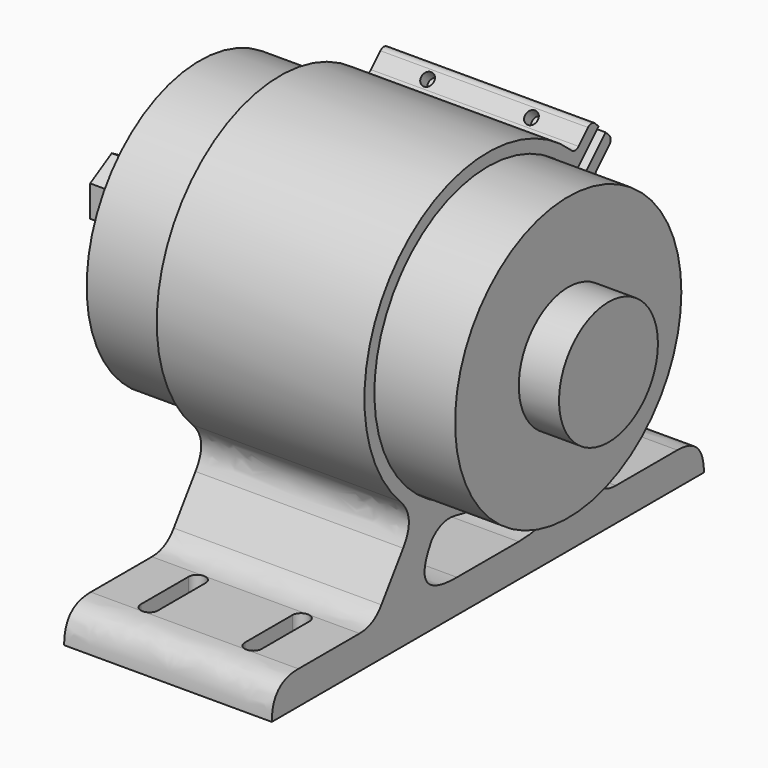
from build123d import *

# Parameters (mm, degrees)
F0_R         = 34.05
F1_DEPTH     = 44.35
F2_R         = 14.875
F3_DEPTH     = 9.7
F4_R         = 6
F5_DEPTH     = 9.55
F6_R         = 12.5
F7_DEPTH     = 2.8
F9_DEPTH     = 8.85
F10_DEPTH    = 25
F11_T1_DEPTH = 50
F11_T3_DEPTH = 90
F13_DEPTH    = 8.0010001
F14_R        = 1.55
F15_DEPTH    = 86.3860158555
F16_R        = 1.5


# Not quite as in the source:
# - a fillet or chamfer that OpenCascade refuses, or shapes differently, is made with other operations: its cross-section is extruded or revolved along the edge and cut away or added


with BuildPart() as f1:
    # F0 (on Right) → F1 (new body, symmetric)
    with BuildSketch(Plane.YZ):
        Circle(F0_R)
    extrude(amount=F1_DEPTH, both=True)

    # F2 (on face) → F3 (join)
    with BuildSketch(Plane.YZ.offset(44.35)):
        Circle(F2_R)
    extrude(amount=F3_DEPTH)

    # F4 (on face) → F5 (join)
    with BuildSketch(Plane(origin=(-44.35, 0, 0), x_dir=(0, -1, 0), z_dir=(-1, 0, 0))):
        Circle(F4_R)
    extrude(amount=F5_DEPTH)


with BuildPart() as f7:
    # F6 (on face) → F7 (new body)
    with BuildSketch(Plane(origin=(-53.9, 0, 0), x_dir=(0, -1, 0), z_dir=(-1, 0, 0))):
        Circle(F6_R)
    extrude(amount=F7_DEPTH)


with BuildPart() as f9:
    # F8 (on face) → F9 (new body)
    with BuildSketch(Plane(origin=(-56.7, 0, 0), x_dir=(0, -1, 0), z_dir=(-1, 0, 0))):
        Polygon((6.5, 3.7527767497), (0, 7.5055534995), (-6.5, 3.7527767497), (-6.5, -3.7527767497), (0, -7.5055534995), (6.5, -3.7527767497), align=None)
    extrude(amount=F9_DEPTH)


with BuildPart() as f10:
    # F0 (on Right) → F10 (new body, symmetric)
    with BuildSketch(Plane.YZ):
        with BuildLine():
            ThreePointArc((28.0146918209, 19.5294531972), (-27.1218147701, -20.7516183363), (26.1756598689, 21.9330191818))
            Line((26.1756598689, 21.9330191818), (33.3400847329, 29.0974440458))
            Line((33.3400847329, 29.0974440458), (31.2187643894, 31.2187643894))
            Line((31.2187643894, 31.2187643894), (26.2690169211, 26.2690169211))
            ThreePointArc((26.2690169211, 26.2690169211), (-28.4585510619, 23.8795596999), (-21.3083646104, -30.4314984453))
            Line((-21.3083646104, -30.4314984453), (-34.415200503, -49.15))
            Line((-34.415200503, -49.15), (-65.0168608087, -49.15))
            Line((-65.0168608087, -49.15), (-65.0168608087, -57.15))
            Line((-65.0168608087, -57.15), (-40.0168608087, -57.15))
            Line((-40.0168608087, -57.15), (40.0168608087, -57.15))
            Line((40.0168608087, -57.15), (65.0168608087, -57.15))
            Line((65.0168608087, -57.15), (65.0168608087, -49.15))
            Line((65.0168608087, -49.15), (34.415200503, -49.15))
            Line((34.415200503, -49.15), (21.3083646104, -30.4314984453))
            ThreePointArc((21.3083646104, -30.4314984453), (36.3368391247, -7.7302407742), (31.8504204749, 19.1225839147))
            Line((31.8504204749, 19.1225839147), (37.5636367015, 24.8358001413))
            Line((37.5636367015, 24.8358001413), (35.4518607172, 26.9666220935))
            Line((35.4518607172, 26.9666220935), (28.0146918209, 19.5294531972))
        make_face()
        with BuildLine():
            Line((14.2552205634, -34.3061391982), (24.6490037929, -49.15))
            Line((24.6490037929, -49.15), (-24.6490037929, -49.15))
            Line((-24.6490037929, -49.15), (-14.2552205634, -34.3061391982))
            ThreePointArc((-14.2552205634, -34.3061391982), (0, -37.15), (14.2552205634, -34.3061391982))
        make_face(mode=Mode.SUBTRACT)
    extrude(amount=F10_DEPTH, both=True)

    # F11: fillet of radius 8 on 10 edges, made by hand

    # F11_s2 → F11_t1 (join)
    with BuildSketch(Plane.YZ.offset(-25)):
        with BuildLine():
            add(Edge.make_bspline(
                [(32.0265205531, -45.7386114908), (34.415200503, -49.15), (38.5797369074, -49.15)],
                knots=[0, 0, 0, 1, 1, 1], degree=2, weights=[1, 1, 1]))
            Line((38.5797369074, -49.15), (34.415200503, -49.15))
            Line((34.415200503, -49.15), (32.0265205531, -45.7386114908))
        make_face()
        with BuildLine():
            add(Edge.make_bspline(
                [(-38.5797369074, -49.15), (-34.415200503, -49.15), (-32.0265205531, -45.7386114908)],
                knots=[0, 0, 0, 1, 1, 1], degree=2, weights=[1, 1, 1]))
            Line((-32.0265205531, -45.7386114908), (-34.415200503, -49.15))
            Line((-34.415200503, -49.15), (-38.5797369074, -49.15))
        make_face()
        with BuildLine():
            add(Edge.make_bspline(
                [(-25.4872127895, -36.3995121427), (-21.650943696, -30.9207520836), (-26.363276693, -26.1744177014)],
                knots=[0, 0, 0, 1, 1, 1], degree=2, weights=[1, 1, 1]))
            ThreePointArc((-26.363276693, -26.1744177014), (-23.930671329, -28.4155849798), (-21.3083646104, -30.4314984453))
            Line((-21.3083646104, -30.4314984453), (-25.4872127895, -36.3995121427))
        make_face()
        with BuildLine():
            add(Edge.make_bspline(
                [(-15.8343631315, -36.5613885092), (-24.6490037929, -49.15), (-9.2811467771, -49.15)],
                knots=[0, 0, 0, 1, 1, 1], degree=2, weights=[1, 1, 1]))
            Line((-9.2811467771, -49.15), (-24.6490037929, -49.15))
            Line((-24.6490037929, -49.15), (-15.8343631315, -36.5613885092))
        make_face()
        with BuildLine():
            add(Edge.make_bspline(
                [(9.2811467771, -49.15), (24.6490037929, -49.15), (15.8343631315, -36.5613885092)],
                knots=[0, 0, 0, 1, 1, 1], degree=2, weights=[1, 1, 1]))
            Line((15.8343631315, -36.5613885092), (24.6490037929, -49.15))
            Line((24.6490037929, -49.15), (9.2811467771, -49.15))
        make_face()
        with BuildLine():
            add(Edge.make_bspline(
                [(17.6631407114, -39.1731535648), (14.4950155025, -34.6486018625), (9.1413884799, -36.0077424544)],
                knots=[0, 0, 0, 1, 1, 1], degree=2, weights=[1, 1, 1]))
            ThreePointArc((9.1413884799, -36.0077424544), (11.7292025343, -35.2497986932), (14.2552205634, -34.3061391982))
            Line((14.2552205634, -34.3061391982), (17.6631407114, -39.1731535648))
        make_face()
        with BuildLine():
            add(Edge.make_bspline(
                [(26.363276693, -26.1744177014), (21.650943696, -30.9207520836), (25.4872127895, -36.3995121427)],
                knots=[0, 0, 0, 1, 1, 1], degree=2, weights=[1, 1, 1]))
            Line((25.4872127895, -36.3995121427), (21.3083646104, -30.4314984453))
            ThreePointArc((21.3083646104, -30.4314984453), (23.930671329, -28.4155849798), (26.363276693, -26.1744177014))
        make_face()
        with BuildLine():
            add(Edge.make_bspline(
                [(-17.6631407114, -39.1731535648), (-14.4950155025, -34.6486018625), (-9.1413884799, -36.0077424544)],
                knots=[0, 0, 0, 1, 1, 1], degree=2, weights=[1, 1, 1]))
            ThreePointArc((-9.1413884799, -36.0077424544), (-11.7292025343, -35.2497986932), (-14.2552205634, -34.3061391982))
            Line((-14.2552205634, -34.3061391982), (-17.6631407114, -39.1731535648))
        make_face()
    extrude(amount=F11_T1_DEPTH)

    # F11_s4 → F11_t3 (cut)
    with BuildSketch(Plane.YZ.offset(-45)):
        with BuildLine():
            add(Edge.make_bspline(
                [(-57.0168608087, -49.15), (-65.0168608087, -49.15), (-65.0168608087, -57.15)],
                knots=[0, 0, 0, 1, 1, 1], degree=2, weights=[1, 1, 1]))
            Line((-65.0168608087, -57.15), (-65.0168608087, -49.15))
            Line((-65.0168608087, -49.15), (-57.0168608087, -49.15))
        make_face()
        with BuildLine():
            add(Edge.make_bspline(
                [(65.0168608087, -57.15), (65.0168608087, -49.15), (57.0168608087, -49.15)],
                knots=[0, 0, 0, 1, 1, 1], degree=2, weights=[1, 1, 1]))
            Line((57.0168608087, -49.15), (65.0168608087, -49.15))
            Line((65.0168608087, -49.15), (65.0168608087, -57.15))
        make_face()
    extrude(amount=F11_T3_DEPTH, mode=Mode.SUBTRACT)

    # F12 (on face) → F13 (cut, through all)
    with BuildSketch(Plane.XY.offset(-49.15)):
        with BuildLine():
            ThreePointArc((-10.45, 54.9668608087), (-11.0504310986, 56.4164297101), (-12.5, 57.0168608087))
            ThreePointArc((-12.5, 57.0168608087), (-13.9495689014, 56.4164297101), (-14.55, 54.9668608087))
            Line((-14.55, 54.9668608087), (-14.55, 40.6297369074))
            ThreePointArc((-14.55, 40.6297369074), (-13.9495689014, 39.180168006), (-12.5, 38.5797369074))
            ThreePointArc((-12.5, 38.5797369074), (-11.0504310986, 39.180168006), (-10.45, 40.6297369074))
            Line((-10.45, 40.6297369074), (-10.45, 54.9668608087))
        make_face()
        with BuildLine():
            ThreePointArc((14.55, 54.9668608087), (13.9495689014, 56.4164297101), (12.5, 57.0168608087))
            ThreePointArc((12.5, 57.0168608087), (11.0504310986, 56.4164297101), (10.45, 54.9668608087))
            Line((10.45, 54.9668608087), (10.45, 40.6297369074))
            ThreePointArc((10.45, 40.6297369074), (11.0504310986, 39.180168006), (12.5, 38.5797369074))
            ThreePointArc((12.5, 38.5797369074), (13.9495689014, 39.180168006), (14.55, 40.6297369074))
            Line((14.55, 40.6297369074), (14.55, 54.9668608087))
        make_face()
        with BuildLine():
            Line((14.55, -54.9668608087), (14.55, -40.6297369074))
            ThreePointArc((14.55, -40.6297369074), (12.5, -38.5797369074), (10.45, -40.6297369074))
            Line((10.45, -40.6297369074), (10.45, -54.9668608087))
            ThreePointArc((10.45, -54.9668608087), (12.5, -57.0168608087), (14.55, -54.9668608087))
        make_face()
        with BuildLine():
            Line((-10.45, -54.9668608087), (-10.45, -40.6297369074))
            ThreePointArc((-10.45, -40.6297369074), (-12.5, -38.5797369074), (-14.55, -40.6297369074))
            Line((-14.55, -40.6297369074), (-14.55, -54.9668608087))
            ThreePointArc((-14.55, -54.9668608087), (-12.5, -57.0168608087), (-10.45, -54.9668608087))
        make_face()
    extrude(amount=-F13_DEPTH, mode=Mode.SUBTRACT)

    # F14 (on face) → F15 (cut, through all)
    with BuildSketch(Plane(origin=(0, 0, 0), x_dir=(1, 0, 0), z_dir=(0, -0.7071067812, 0.7071067812))):
        with Locations((-12.5, 40.65)):
            Circle(F14_R)
        with Locations((12.5, 40.65)):
            Circle(F14_R)
    extrude(amount=-F15_DEPTH, mode=Mode.SUBTRACT)

    # F16
    f16_edges = [f10.edges().sort_by_distance(p)[0] for p in [
        (0, 31.218764, 31.218764),
        (0, 37.563637, 24.8358),
        (0, 31.85042, 19.122584),
        (0, 26.269017, 26.269017),
    ]]
    fillet(f16_edges, radius=F16_R)


solid = Compound([f1.part, f7.part, f9.part, f10.part])
